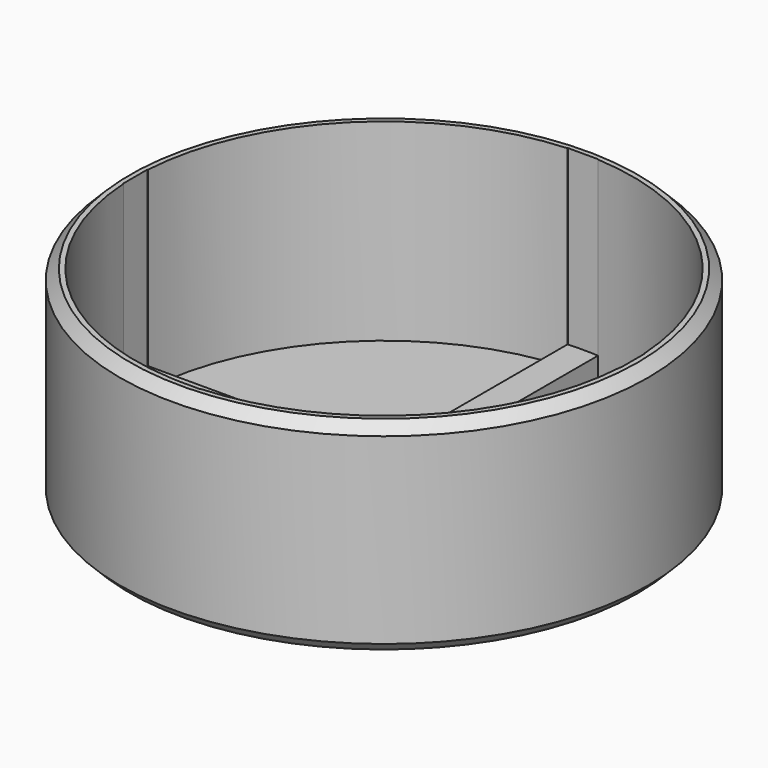
from build123d import *

# Parameters (mm, degrees)
F0_W     = 3.81
F0_H     = 3.81
F0_R     = 0.508
F1_DEPTH = 3.81
F2_DEPTH = 1.27
F4_R     = 0.9525
F5_DEPTH = 25.4
F0_R_2   = 33.02
F6_DEPTH = 25.4
F7_SIZE  = 1.27


# Not quite as in the source:
# - a feature names something its author has since deleted; it is built from what else it names


with BuildPart() as f1:
    # F0 (on Top) → F1 (new body)
    with BuildSketch(Plane.XY):
        Rectangle(F0_W, F0_H)
        Circle(F0_R, mode=Mode.SUBTRACT)
        with BuildLine():
            ThreePointArc((31.056628922, -1.905), (31.1004038069, -0.9529470319), (31.115, 0))
            ThreePointArc((31.115, 0), (31.1004038069, 0.9529470319), (31.056628922, 1.905))
            Line((31.056628922, 1.905), (1.905, 1.905))
            Line((1.905, 1.905), (1.905, -1.905))
            Line((1.905, -1.905), (31.056628922, -1.905))
        make_face()
        with BuildLine():
            ThreePointArc((0, -31.115), (0.9529470319, -31.1004038069), (1.905, -31.056628922))
            Line((1.905, -31.056628922), (1.905, -1.905))
            Line((1.905, -1.905), (-1.905, -1.905))
            Line((-1.905, -1.905), (-1.905, -31.056628922))
            ThreePointArc((-1.905, -31.056628922), (-0.9529470319, -31.1004038069), (0, -31.115))
        make_face()
        with BuildLine():
            Line((-1.905, -1.905), (-1.905, 1.905))
            Line((-1.905, 1.905), (-31.056628922, 1.905))
            ThreePointArc((-31.056628922, 1.905), (-31.1004038069, 0.9529470319), (-31.115, 0))
            ThreePointArc((-31.115, 0), (-31.1004038069, -0.9529470319), (-31.056628922, -1.905))
            Line((-31.056628922, -1.905), (-1.905, -1.905))
        make_face()
        with BuildLine():
            Line((1.905, 1.905), (1.905, 31.056628922))
            ThreePointArc((1.905, 31.056628922), (0.9529470319, 31.1004038069), (0, 31.115))
            ThreePointArc((0, 31.115), (-0.9529470319, 31.1004038069), (-1.905, 31.056628922))
            Line((-1.905, 31.056628922), (-1.905, 1.905))
            Line((-1.905, 1.905), (1.905, 1.905))
        make_face()
    extrude(amount=F1_DEPTH)

    # F0 (on Top) → F2 (join)
    with BuildSketch(Plane.XY):
        with BuildLine():
            Line((1.905, 1.905), (1.905, 31.056628922))
            ThreePointArc((1.905, 31.056628922), (0.9529470319, 31.1004038069), (0, 31.115))
            ThreePointArc((0, 31.115), (-0.9529470319, 31.1004038069), (-1.905, 31.056628922))
            Line((-1.905, 31.056628922), (-1.905, 1.905))
            Line((-1.905, 1.905), (1.905, 1.905))
        make_face()
        with BuildLine():
            ThreePointArc((0, -31.115), (0.9529470319, -31.1004038069), (1.905, -31.056628922))
            Line((1.905, -31.056628922), (1.905, -1.905))
            Line((1.905, -1.905), (-1.905, -1.905))
            Line((-1.905, -1.905), (-1.905, -31.056628922))
            ThreePointArc((-1.905, -31.056628922), (-0.9529470319, -31.1004038069), (0, -31.115))
        make_face()
        with BuildLine():
            Line((-31.056628922, 1.905), (-1.905, 1.905))
            Line((-1.905, 1.905), (-1.905, 31.056628922))
            ThreePointArc((-1.905, 31.056628922), (-22.0016274966, 22.0016274966), (-31.056628922, 1.905))
        make_face()
        with BuildLine():
            Line((-1.905, -31.056628922), (-1.905, -1.905))
            Line((-1.905, -1.905), (-31.056628922, -1.905))
            ThreePointArc((-31.056628922, -1.905), (-22.0016274966, -22.0016274966), (-1.905, -31.056628922))
        make_face()
        with BuildLine():
            Line((1.905, 1.905), (31.056628922, 1.905))
            ThreePointArc((31.056628922, 1.905), (22.0016274966, 22.0016274966), (1.905, 31.056628922))
            Line((1.905, 31.056628922), (1.905, 1.905))
        make_face()
        with BuildLine():
            ThreePointArc((1.905, -31.056628922), (22.0016274966, -22.0016274966), (31.056628922, -1.905))
            Line((31.056628922, -1.905), (1.905, -1.905))
            Line((1.905, -1.905), (1.905, -31.056628922))
        make_face()
    extrude(amount=F2_DEPTH)

    # F4 (on offset) → F5 (cut)
    with BuildSketch(Plane.YZ.offset(-5.08)):
        Circle(F4_R)
    extrude(amount=-F5_DEPTH, mode=Mode.SUBTRACT)


with BuildPart() as f6:
    # F0 (on Top) → F6 (new body)
    with BuildSketch(Plane.XY):
        Circle(F0_R_2)
        with BuildLine():
            Line((31.115, 1.905), (31.115, 0))
            Line((31.115, 0), (31.115, -1.905))
            Line((31.115, -1.905), (31.056628922, -1.905))
            ThreePointArc((31.056628922, -1.905), (22.0016274966, -22.0016274966), (1.905, -31.056628922))
            Line((1.905, -31.056628922), (1.905, -31.115))
            Line((1.905, -31.115), (0, -31.115))
            ThreePointArc((0, -31.115), (-0.9529470319, -31.1004038069), (-1.905, -31.056628922))
            ThreePointArc((-1.905, -31.056628922), (-22.0016274966, -22.0016274966), (-31.056628922, -1.905))
            Line((-31.056628922, -1.905), (-31.115, -1.905))
            Line((-31.115, -1.905), (-31.115, 0))
            Line((-31.115, 0), (-31.115, 1.905))
            Line((-31.115, 1.905), (-31.056628922, 1.905))
            ThreePointArc((-31.056628922, 1.905), (-22.0016274966, 22.0016274966), (-1.905, 31.056628922))
            Line((-1.905, 31.056628922), (-1.905, 31.115))
            Line((-1.905, 31.115), (0, 31.115))
            Line((0, 31.115), (1.905, 31.115))
            Line((1.905, 31.115), (1.905, 31.056628922))
            ThreePointArc((1.905, 31.056628922), (22.0016274966, 22.0016274966), (31.056628922, 1.905))
            Line((31.056628922, 1.905), (31.115, 1.905))
        make_face(mode=Mode.SUBTRACT)
    extrude(amount=F6_DEPTH)

    # F7
    f7_edges = [f6.edges().sort_by_distance(p)[0] for p in [
        (-33.02, 0, 25.4),
        (-33.02, 0, 0),
    ]]
    chamfer(f7_edges, length=F7_SIZE)


solid = Compound([f1.part, f6.part])
